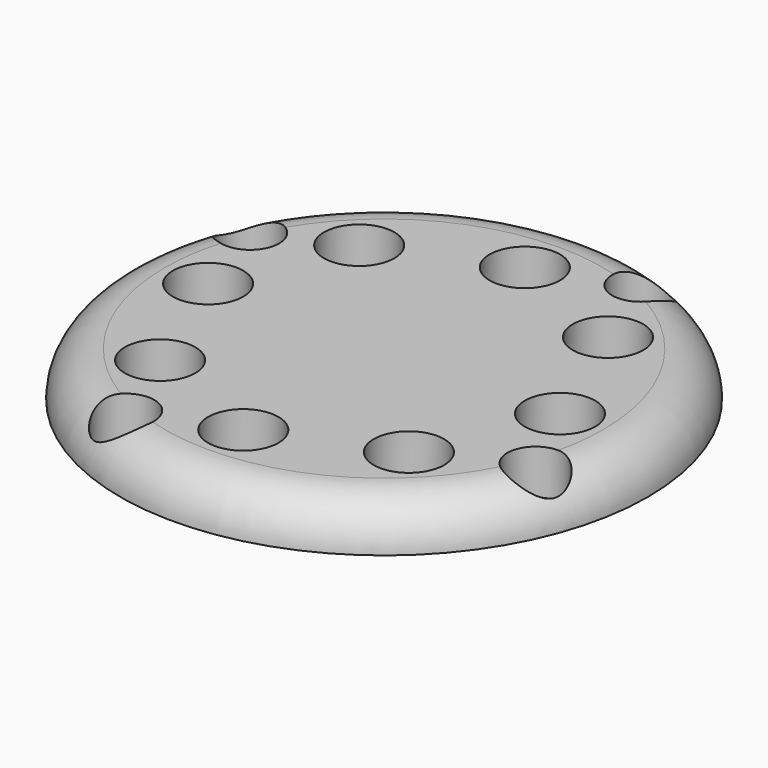
from build123d import *

# Parameters (mm, degrees)
F0_R     = 75
F0_R_2   = 8.1306454005
F0_R_3   = 10
F0_R_4   = 8.004103626
F0_R_5   = 8.2498069198
F0_R_6   = 7.9610699334
F1_DEPTH = 12.7


# Not quite as in the source:
# - a fillet or chamfer that OpenCascade refuses, or shapes differently, is made with other operations: its cross-section is extruded or revolved along the edge and cut away or added
# - the program builds the solid bodies; features that only make, move or delete a surface that nothing else refers to are left out


with BuildPart() as f1:
    # F0 (on Top) → F1 (new body)
    with BuildSketch(Plane.XY):
        Circle(F0_R)
        with Locations((-26.2292288244, -59.023771435)):
            Circle(F0_R_2, mode=Mode.SUBTRACT)
        with Locations((-50, -0.0119686127)):
            Circle(F0_R_3, mode=Mode.SUBTRACT)
        with Locations((-35.3553390593, -35.367307672)):
            Circle(F0_R_3, mode=Mode.SUBTRACT)
        with Locations((0, -50.0119686127)):
            Circle(F0_R_3, mode=Mode.SUBTRACT)
        with Locations((35.3553390593, -35.367307672)):
            Circle(F0_R_3, mode=Mode.SUBTRACT)
        with Locations((60.637563467, -22.0063943416)):
            Circle(F0_R_4, mode=Mode.SUBTRACT)
        with Locations((50, -0.0119686127)):
            Circle(F0_R_3, mode=Mode.SUBTRACT)
        with Locations((-58.0026507378, 24.9211471528)):
            Circle(F0_R_5, mode=Mode.SUBTRACT)
        with Locations((-35.3553390593, 35.3433704467)):
            Circle(F0_R_3, mode=Mode.SUBTRACT)
        with Locations((35.3553390593, 35.3433704467)):
            Circle(F0_R_3, mode=Mode.SUBTRACT)
        with Locations((0, 49.9880313873)):
            Circle(F0_R_3, mode=Mode.SUBTRACT)
        with Locations((25.3583583981, 59.3152455986)):
            Circle(F0_R_6, mode=Mode.SUBTRACT)
    extrude(amount=F1_DEPTH)

    # F2: fillet of radius 12.7 on 1 edges, made by hand

    # F2_s1 → F2_t2 (revolve, cut)
    with BuildSketch(Plane.XZ):
        with BuildLine():
            ThreePointArc((75, 0), (71.2802561211, 8.9802561211), (62.3, 12.7))
            Line((62.3, 12.7), (75, 12.7))
            Line((75, 12.7), (75, 0))
        make_face()
    revolve(axis=Axis((0, 0, 12.7), (0, 0, 1)), mode=Mode.SUBTRACT)


solid = f1.part
